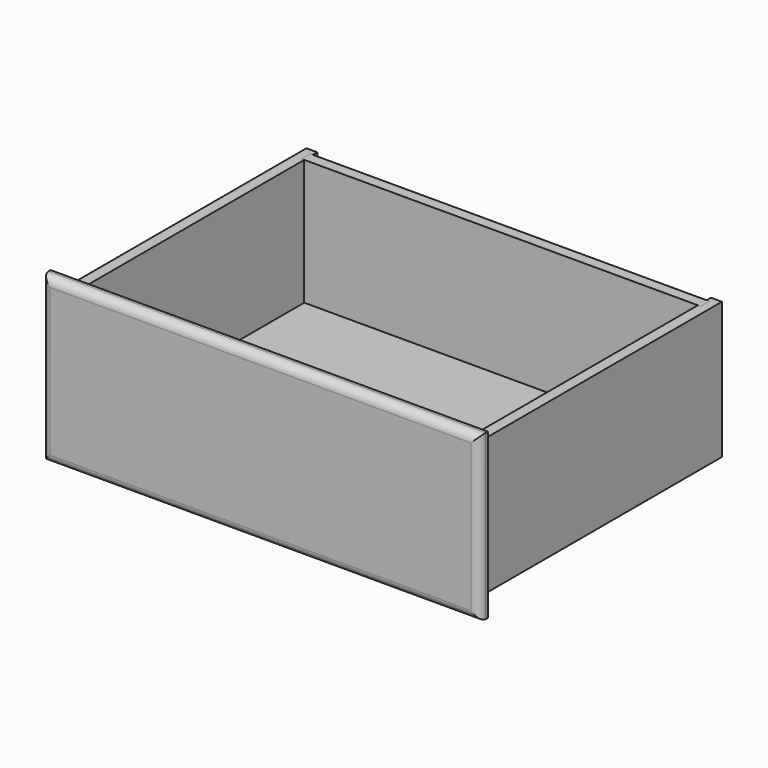
from build123d import *

# Parameters (mm, degrees)
F0_W      = 508
F0_H      = 190.5
F1_DEPTH  = 12.7
F2_R      = 9.525
F3_W      = 457.2
F3_H      = 158.75
F4_DEPTH  = 12.7
F5_W      = 12.7
F5_H      = 158.75
F6_DEPTH  = 355.6
F7_W      = 12.7
F7_H      = 158.75
F8_DEPTH  = 355.6
F9_W      = 3.175
F9_H      = 12.7
F10_DEPTH = 174.626
F11_W     = 3.175
F11_H     = 12.7
F12_DEPTH = 174.626
F14_DEPTH = 158.75
F15_W     = 463.55
F15_H     = 6.35
F16_DEPTH = 3.175
F17_W     = 336.55
F17_H     = 6.35
F18_DEPTH = 3.175
F20_DEPTH = 3.175
F21_W     = 457.2
F21_H     = 6.35
F22_DEPTH = 3.175
F23_W     = 463.55
F23_H     = 327.025
F24_DEPTH = 6.35


# Not quite as in the source:
# - a feature names something its author has since deleted; it is built from what else it names


with BuildPart() as f1:
    # F0 (on Front) → F1 (new body)
    with BuildSketch(Plane.XZ):
        with Locations((-8.8439956307, -13.6189054852)):
            Rectangle(F0_W, F0_H)
    extrude(amount=F1_DEPTH)

    # F2
    f2_edges = [f1.edges().sort_by_distance(p)[0] for p in [
        (-8.843996, -12.7, 81.631095),
        (-262.843996, -12.7, -13.618905),
        (-8.843996, -12.7, -108.868905),
        (245.156004, -12.7, -13.618905),
    ]]
    fillet(f2_edges, radius=F2_R)

    # F3 (on face) → F4 (join)
    with BuildSketch(Plane(origin=(0, 0, 0), x_dir=(-1, 0, 0), z_dir=(0, 1, 0))):
        with Locations((8.8439956307, -13.6189054852)):
            Rectangle(F3_W, F3_H)
    extrude(amount=F4_DEPTH)

    # F21 (on face) → F22 (cut)
    with BuildSketch(Plane(origin=(0, 12.7, 0), x_dir=(-1, 0, 0), z_dir=(0, 1, 0))):
        with Locations((8.8439956307, -83.4689054852)):
            Rectangle(F21_W, F21_H)
    extrude(amount=-F22_DEPTH, mode=Mode.SUBTRACT)


with BuildPart() as f6:
    # F5 (on face) → F6 (new body)
    with BuildSketch(Plane(origin=(0, 0, 0), x_dir=(-1, 0, 0), z_dir=(0, 1, 0))):
        with Locations((-226.1060043693, -13.6189054852)):
            Rectangle(F5_W, F5_H)
    extrude(amount=F6_DEPTH)

    # F11 (on face) → F12 (cut, through all)
    with BuildSketch(Plane.XY.offset(65.7560945148)):
        with Locations((221.3435043693, 342.9)):
            Rectangle(F11_W, F11_H)
    extrude(amount=-F12_DEPTH, mode=Mode.SUBTRACT)

    # F17 (on face) → F18 (cut)
    with BuildSketch(Plane(origin=(219.7560043693, 0, 0), x_dir=(0, -1, 0), z_dir=(-1, 0, 0))):
        with Locations((-168.275, -83.4689054852)):
            Rectangle(F17_W, F17_H)
    extrude(amount=-F18_DEPTH, mode=Mode.SUBTRACT)


with BuildPart() as f8:
    # F7 (on face) → F8 (new body)
    with BuildSketch(Plane(origin=(0, 0, 0), x_dir=(-1, 0, 0), z_dir=(0, 1, 0))):
        with Locations((243.7939956307, -13.6189054852)):
            Rectangle(F7_W, F7_H)
    extrude(amount=F8_DEPTH)

    # F9 (on face) → F10 (cut, through all)
    with BuildSketch(Plane.XY.offset(65.7560945148)):
        with Locations((-239.0314956307, 342.9)):
            Rectangle(F9_W, F9_H)
    extrude(amount=-F10_DEPTH, mode=Mode.SUBTRACT)

    # F19 (on face) → F20 (cut)
    with BuildSketch(Plane.YZ.offset(-237.4439956307)):
        Polygon((0, -85.2191895247), (0, -86.6439054852), (5.2507231012, -86.6439054852), (336.55, -86.6439054852), (336.55, -80.2939054852), (0, -80.2939054852), align=None)
    extrude(amount=-F20_DEPTH, mode=Mode.SUBTRACT)


with BuildPart() as f14:
    # F13 (on face) → F14 (new body)
    with BuildSketch(Plane.XY.offset(65.7560945148)):
        Polygon((-237.4439956307, 349.25), (-240.6189956307, 349.25), (-240.6189956307, 336.55), (-237.4439956307, 336.55), (222.9310043693, 336.55), (222.9310043693, 349.25), align=None)
    extrude(amount=-F14_DEPTH)

    # F15 (on face) → F16 (cut)
    with BuildSketch(Plane.XZ.offset(-336.55)):
        with Locations((-8.8439956307, -83.4689054852)):
            Rectangle(F15_W, F15_H)
    extrude(amount=-F16_DEPTH, mode=Mode.SUBTRACT)


with BuildPart() as f24:
    # F23 (on face) → F24 (new body)
    with BuildSketch(Plane.XY.offset(-86.6439054852)):
        with Locations((-8.8439956307, 173.0375)):
            Rectangle(F23_W, F23_H)
    extrude(amount=F24_DEPTH)


solid = Compound([f1.part, f6.part, f8.part, f14.part, f24.part])
